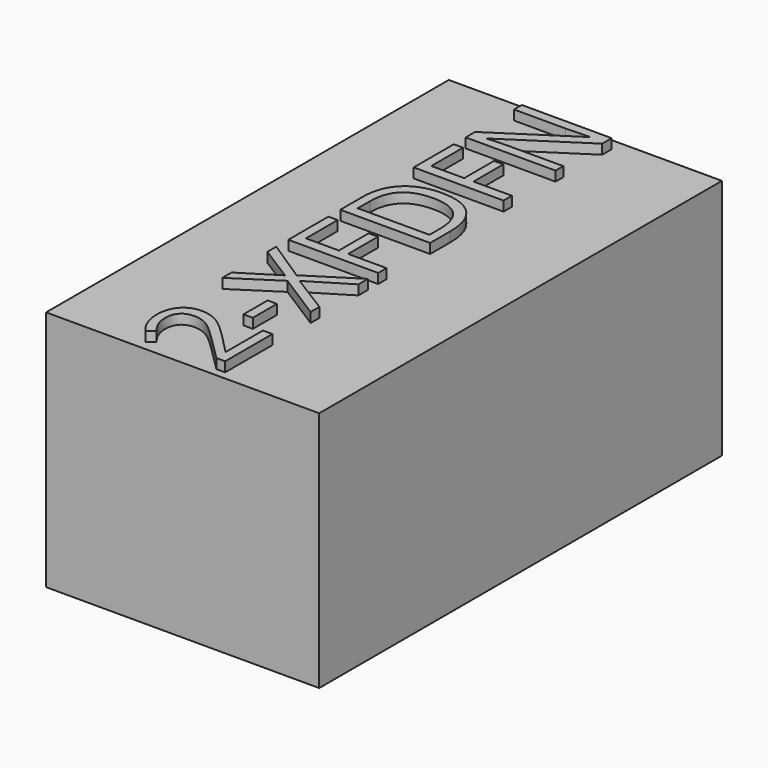
from build123d import *

# Parameters (mm, degrees)
F0_W         = 0.254
F0_H         = 0.15494
F1_DEPTH     = 0.01524
F2_W         = 0.3556
F2_H         = 0.65532
F3_DEPTH     = 0.31496
F4_TEXT_SIZE = 0.1638709677
F5_DEPTH     = 0.0127


# Not quite as in the source:
# - Text() gives the source's letters only with a copy of the font that has no kerning and outlines rounded to 1/6400 em; it was checked with that copy


with BuildPart() as f1:
    # F0 (on Top) → F1 (new body)
    with BuildSketch(Plane.XY):
        with Locations((0, 0.19939)):
            Rectangle(F0_W, F0_H)
    extrude(amount=F1_DEPTH)


with BuildPart() as f1b:
    # F0 (on Top) → F1, piece 2 (new body)
    with BuildSketch(Plane.XY):
        with Locations((0, -0.19939)):
            Rectangle(F0_W, F0_H)
    extrude(amount=F1_DEPTH)


with BuildPart() as f3:
    # F2 (on face) → F3 (new body)
    with BuildSketch(Plane.XY.offset(0.01524)):
        Rectangle(F2_W, F2_H)
    extrude(amount=F3_DEPTH)

    # F4 (on face) → F5 (join)
    with BuildSketch(Plane.XY.offset(0.3302)):
        with Locations(Location((0.0468670968, -0.32512), (0, 0, 90))):
            Text('2-XFDFN', F4_TEXT_SIZE, font='Open Sans', text_align=(TextAlign.LEFT, TextAlign.BOTTOM))
    extrude(amount=F5_DEPTH)


solid = Compound([f1.part, f1b.part, f3.part])
